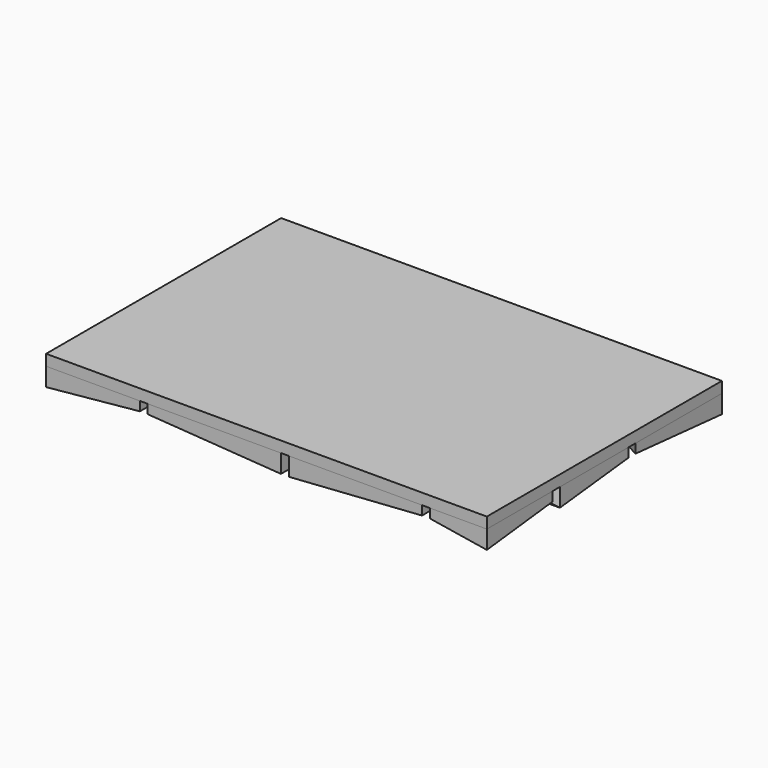
from build123d import *

# Parameters (mm, degrees)
F1_DEPTH = 1.905
F3_DEPTH = 6.35
F5_W     = 3.1199518736
F5_H     = 3.175
F6_DEPTH = 152.401
F7_DEPTH = 101.601


with BuildPart() as f1:
    # F0 (on Top) → F1 (new body, symmetric)
    with BuildSketch(Plane.XY):
        with BuildLine():
            Line((86.9781998813, 49.6921139163), (-51.5174866416, 49.6921139163))
            ThreePointArc((-51.5174866416, 49.6921139163), (-51.0547363677, 47.8612091542), (-50.8990761846, 45.9791570902))
            ThreePointArc((-50.8990761846, 45.9791570902), (-55.4230496017, 36.8586861927), (-65.4218001187, 34.9418364415))
            Line((-65.4218001187, 34.9418364415), (-65.4218001187, -51.9078860837))
            Line((-65.4218001187, -51.9078860837), (86.9781998813, -51.9078860837))
            Line((86.9781998813, -51.9078860837), (86.9781998813, 49.6921139163))
        make_face()
        with BuildLine():
            Line((-51.5174866416, 49.6921139163), (-65.4218001187, 49.6921139163))
            Line((-65.4218001187, 49.6921139163), (-65.4218001187, 34.9418364415))
            ThreePointArc((-65.4218001187, 34.9418364415), (-55.4230496017, 36.8586861927), (-50.8990761846, 45.9791570902))
            ThreePointArc((-50.8990761846, 45.9791570902), (-51.0547363677, 47.8612091542), (-51.5174866416, 49.6921139163))
        make_face()
    extrude(amount=F1_DEPTH, both=True)


with BuildPart() as f3:
    # F2 (on face) → F3 (new body)
    with BuildSketch(Plane(origin=(0, 0, -1.905), x_dir=(1, 0, 0), z_dir=(0, 0, -1))):
        Polygon((-56.0116855077, 21.531348115), (-32.9786642982, 34.8294691105), (-32.9786642982, 48.127590106), (-32.9786642982, 51.9078860837), (-65.4218001187, 51.9078860837), (-65.4218001187, 26.9642803188), align=None)
    extrude(amount=F3_DEPTH)


with BuildPart() as f3b:
    # F2 (on face) → F3, piece 2 (new body)
    with BuildSketch(Plane(origin=(0, 0, -1.905), x_dir=(1, 0, 0), z_dir=(0, 0, -1))):
        Polygon((-56.7653295392, 18.8582386622), (-65.4218001187, 23.8560542815), (-65.4218001187, -12.7358189481), (-56.7653295392, -7.7380033289), align=None)
    extrude(amount=F3_DEPTH)


with BuildPart() as f3c:
    # F2 (on face) → F3, piece 3 (new body)
    with BuildSketch(Plane(origin=(0, 0, -1.905), x_dir=(1, 0, 0), z_dir=(0, 0, -1))):
        Polygon((-55.372, -10.0535160179), (-65.4218001187, -15.8557708218), (-65.4218001187, -49.6921139163), (-32.3389787906, -49.6921139163), (-32.3389787906, -23.3516370134), align=None)
    extrude(amount=F3_DEPTH)


with BuildPart() as f3d:
    # F2 (on face) → F3, piece 4 (new body)
    with BuildSketch(Plane(origin=(0, 0, -1.905), x_dir=(1, 0, 0), z_dir=(0, 0, -1))):
        Polygon((-7.9973295392, 18.8582386622), (-31.0303507486, 32.1563596577), (-54.0633719581, 18.8582386622), (-54.0633719581, -7.7380033289), (-31.0303507486, -21.0361243244), (-7.9973295392, -7.7380033289), align=None)
    extrude(amount=F3_DEPTH)


with BuildPart() as f3e:
    # F2 (on face) → F3, piece 5 (new body)
    with BuildSketch(Plane(origin=(0, 0, -1.905), x_dir=(1, 0, 0), z_dir=(0, 0, -1))):
        Polygon((-30.2767067171, 51.9078860837), (-30.2767067171, 48.127590106), (-30.2767067171, 34.8294691105), (-7.2436855077, 21.531348115), (15.7893357018, 34.8294691105), (15.7893357018, 51.9078860837), align=None)
    extrude(amount=F3_DEPTH)


with BuildPart() as f3f:
    # F2 (on face) → F3, piece 6 (new body)
    with BuildSketch(Plane(origin=(0, 0, -1.905), x_dir=(1, 0, 0), z_dir=(0, 0, -1))):
        Polygon((40.7706704608, 18.8582386622), (17.7376492514, 32.1563596577), (-5.2953719581, 18.8582386622), (-5.2953719581, -7.7380033289), (17.7376492514, -21.0361243244), (40.7706704608, -7.7380033289), align=None)
    extrude(amount=F3_DEPTH)


with BuildPart() as f3g:
    # F2 (on face) → F3, piece 7 (new body)
    with BuildSketch(Plane(origin=(0, 0, -1.905), x_dir=(1, 0, 0), z_dir=(0, 0, -1))):
        Polygon((-29.6370212094, -23.3516370134), (-29.6370212094, -49.6921139163), (16.4290212094, -49.6921139163), (16.4290212094, -23.3516370134), (-6.604, -10.0535160179), align=None)
    extrude(amount=F3_DEPTH)


with BuildPart() as f3h:
    # F2 (on face) → F3, piece 8 (new body)
    with BuildSketch(Plane(origin=(0, 0, -1.905), x_dir=(1, 0, 0), z_dir=(0, 0, -1))):
        Polygon((19.1309787906, -23.3516370134), (19.1309787906, -49.6921139163), (65.1970212094, -49.6921139163), (65.1970212094, -23.3516370134), (42.164, -10.0535160179), align=None)
    extrude(amount=F3_DEPTH)


with BuildPart() as f3i:
    # F2 (on face) → F3, piece 9 (new body)
    with BuildSketch(Plane(origin=(0, 0, -1.905), x_dir=(1, 0, 0), z_dir=(0, 0, -1))):
        Polygon((86.9781998813, -9.2162917072), (86.9781998813, 20.3365270405), (66.5056492514, 32.1563596577), (43.4726280419, 18.8582386622), (43.4726280419, -7.7380033289), (66.5056492514, -21.0361243244), align=None)
    extrude(amount=F3_DEPTH)


with BuildPart() as f3j:
    # F2 (on face) → F3, piece 10 (new body)
    with BuildSketch(Plane(origin=(0, 0, -1.905), x_dir=(1, 0, 0), z_dir=(0, 0, -1))):
        Polygon((64.5573357018, 51.9078860837), (18.4912932829, 51.9078860837), (18.4912932829, 34.8294691105), (41.5243144923, 21.531348115), (64.5573357018, 34.8294691105), align=None)
    extrude(amount=F3_DEPTH)


with BuildPart() as f3k:
    # F2 (on face) → F3, piece 11 (new body)
    with BuildSketch(Plane(origin=(0, 0, -1.905), x_dir=(1, 0, 0), z_dir=(0, 0, -1))):
        Polygon((86.9781998813, 51.9078860837), (67.2592932829, 51.9078860837), (67.2592932829, 34.8294691105), (86.9781998813, 23.4447530778), align=None)
    extrude(amount=F3_DEPTH)


with BuildPart() as f3l:
    # F2 (on face) → F3, piece 12 (new body)
    with BuildSketch(Plane(origin=(0, 0, -1.905), x_dir=(1, 0, 0), z_dir=(0, 0, -1))):
        Polygon((67.8989787906, -23.3516370134), (67.8989787906, -49.6921139163), (86.9781998813, -49.6921139163), (86.9781998813, -12.3362435808), align=None)
    extrude(amount=F3_DEPTH)


with BuildPart() as f6_tool:
    # F5 (on face) → F6 (new body, through all)
    with BuildSketch(Plane.YZ.offset(86.9781998813)):
        Polygon((21.0361243244, -8.255), (49.6921139163, -8.255), (12.3362435808, -5.08), (12.3362435808, -8.255), align=None)
        Polygon((9.2162917072, -8.255), (9.2162917072, -5.08), (-20.3365270405, -8.255), align=None)
        Polygon((-23.4447530778, -8.255), (-23.4447530778, -5.08), (-51.9078860837, -8.255), (-32.1563596577, -8.255), align=None)
        with Locations((10.776267644, -6.6675)):
            Rectangle(F5_W, F5_H)
        Polygon((-23.4447530778, -8.255), (-20.3365270405, -8.255), (-23.4447530778, -5.08), align=None)
    extrude(amount=-F6_DEPTH)


with BuildPart() as f3i_1:
    add(f3i.part)

    # F6: cut by f6_tool
    add(f6_tool.part, mode=Mode.SUBTRACT)


with BuildPart() as f3k_1:
    add(f3k.part)

    # F6: cut by f6_tool
    add(f6_tool.part, mode=Mode.SUBTRACT)


with BuildPart() as f3l_1:
    add(f3l.part)

    # F6: cut by f6_tool
    add(f6_tool.part, mode=Mode.SUBTRACT)


with BuildPart() as f7_tool:
    # F4 (on face) → F7 (new body, through all)
    with BuildSketch(Plane.XZ.offset(51.9078860837)):
        Polygon((67.2592932829, -8.255), (86.9781998813, -8.255), (67.2592932829, -5.08), align=None)
        Polygon((43.4726280419, -8.255), (64.5573357018, -8.255), (64.5573357018, -5.08), (18.4912932829, -8.255), (40.7706704608, -8.255), align=None)
        Polygon((-5.2953719581, -8.255), (15.7893357018, -8.255), (-30.2767067171, -5.08), (-30.2767067171, -8.255), align=None)
        Polygon((-32.9786642982, -5.08), (-65.4218001187, -8.255), (-32.9786642982, -8.255), align=None)
    extrude(amount=-F7_DEPTH)


with BuildPart() as f3_1:
    add(f3.part)

    # F7: cut by f7_tool
    add(f7_tool.part, mode=Mode.SUBTRACT)


with BuildPart() as f3e_1:
    add(f3e.part)

    # F7: cut by f7_tool
    add(f7_tool.part, mode=Mode.SUBTRACT)


with BuildPart() as f3j_1:
    add(f3j.part)

    # F7: cut by f7_tool
    add(f7_tool.part, mode=Mode.SUBTRACT)


with BuildPart() as f3k_2:
    add(f3k_1.part)

    # F7: cut by f7_tool
    add(f7_tool.part, mode=Mode.SUBTRACT)


solid = Compound([f1.part, f3b.part, f3c.part, f3d.part, f3f.part, f3g.part, f3h.part, f3i_1.part, f3l_1.part, f3_1.part, f3e_1.part, f3j_1.part, f3k_2.part])
